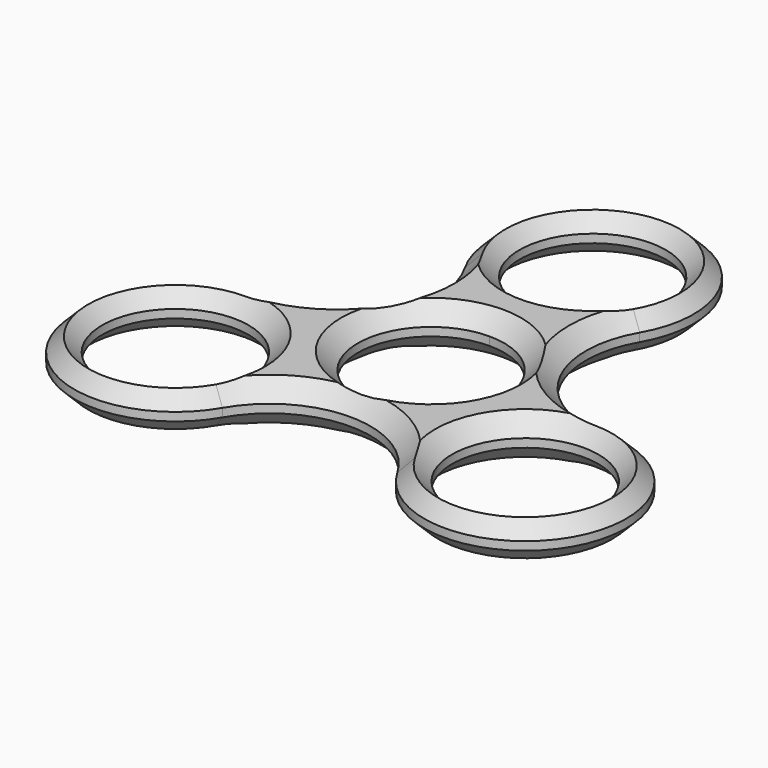
from build123d import *

# Parameters (mm, degrees)
F0_R         = 11.049
F1_DEPTH     = 6.35
F2_T2_ANGLE  = 120
F2_T4_ANGLE  = 240
F2_T6_ANGLE  = 120
F2_T8_ANGLE  = 240
F2_T10_ANGLE = 120
F2_T12_ANGLE = 240
F2_T22_ANGLE = 120
F2_T24_ANGLE = 240
F2_T26_ANGLE = 120
F2_T28_ANGLE = 240
F2_T30_ANGLE = 120
F2_T32_ANGLE = 240


# Not quite as in the source:
# - a fillet or chamfer that OpenCascade refuses, or shapes differently, is made with other operations: its cross-section is extruded or revolved along the edge and cut away or added


with BuildPart() as f1:
    # F0 (on Top) → F1 (new body)
    with BuildSketch(Plane.XY):
        with BuildLine():
            ThreePointArc((26.3964543073, 0), (13.1982271537, 7.62), (13.1982271537, 22.86))
            ThreePointArc((13.1982271537, 22.86), (0, 45.72), (-13.1982271537, 22.86))
            ThreePointArc((-13.1982271537, 22.86), (-13.1982271537, 7.62), (-26.3964543073, 0))
            ThreePointArc((-26.3964543073, 0), (-39.594681461, -22.86), (-13.1982271537, -22.86))
            ThreePointArc((-13.1982271537, -22.86), (0, -15.24), (13.1982271537, -22.86))
            ThreePointArc((13.1982271537, -22.86), (39.594681461, -22.86), (26.3964543073, 0))
        make_face()
        with Locations((-26.3964543073, -15.24)):
            Circle(F0_R, mode=Mode.SUBTRACT)
        with Locations((26.3964543073, -15.24)):
            Circle(F0_R, mode=Mode.SUBTRACT)
        with BuildLine():
            ThreePointArc((0, 11.049), (7.8128228253, 7.8128228253), (11.049, 0))
            ThreePointArc((11.049, 0), (-7.8128228253, -7.8128228253), (0, 11.049))
        make_face(mode=Mode.SUBTRACT)
        with Locations((0, 30.48)):
            Circle(F0_R, mode=Mode.SUBTRACT)
    extrude(amount=F1_DEPTH)

    # F2: chamfer of 2.54 on 20 edges, made by hand

    # F2_s1 → F2_t2 (revolve, cut)
    with BuildSketch(Plane.YZ.offset(26.3964543073)):
        Polygon((0, 3.81), (-2.54, 6.35), (0, 6.35), align=None)
    revolve(axis=Axis((26.3964543073, 15.24, 6.35), (0, 0, -1)), revolution_arc=F2_T2_ANGLE, mode=Mode.SUBTRACT)

    # F2_s3 → F2_t4 (revolve, cut)
    with BuildSketch(Plane(origin=(13.1982271537, 22.86, 0), x_dir=(0, 0, 1), z_dir=(-0.5, -0.8660254038, 0))):
        Polygon((6.35, 2.54), (3.81, 0), (6.35, 0), align=None)
    revolve(axis=Axis((0, 30.48, 6.35), (0, 0, 1)), revolution_arc=F2_T4_ANGLE, mode=Mode.SUBTRACT)

    # F2_s5 → F2_t6 (revolve, cut)
    with BuildSketch(Plane(origin=(-13.1982271537, 22.86, 0), x_dir=(0, 0, 1), z_dir=(-0.5, 0.8660254038, 0))):
        Polygon((6.35, 2.54), (3.81, 0), (6.35, 0), align=None)
    revolve(axis=Axis((-26.3964543073, 15.24, 6.35), (0, 0, -1)), revolution_arc=F2_T6_ANGLE, mode=Mode.SUBTRACT)

    # F2_s7 → F2_t8 (revolve, cut)
    with BuildSketch(Plane.YZ.offset(-26.3964543073)):
        Polygon((-2.54, 6.35), (0, 3.81), (0, 6.35), align=None)
    revolve(axis=Axis((-26.3964543073, -15.24, 6.35), (0, 0, 1)), revolution_arc=F2_T8_ANGLE, mode=Mode.SUBTRACT)

    # F2_s9 → F2_t10 (revolve, cut)
    with BuildSketch(Plane(origin=(-13.1982271537, -22.86, 0), x_dir=(0, 0, 1), z_dir=(-0.5, -0.8660254038, 0))):
        Polygon((6.35, 2.54), (3.81, 0), (6.35, 0), align=None)
    revolve(axis=Axis((0, -30.48, 6.35), (0, 0, -1)), revolution_arc=F2_T10_ANGLE, mode=Mode.SUBTRACT)

    # F2_s11 → F2_t12 (revolve, cut)
    with BuildSketch(Plane(origin=(13.1982271537, -22.86, 0), x_dir=(0, 0, 1), z_dir=(-0.5, 0.8660254038, 0))):
        Polygon((6.35, 2.54), (3.81, 0), (6.35, 0), align=None)
    revolve(axis=Axis((26.3964543073, -15.24, 6.35), (0, 0, 1)), revolution_arc=F2_T12_ANGLE, mode=Mode.SUBTRACT)

    # F2_s13 → F2_t14 (revolve, cut)
    with BuildSketch(Plane.XZ.offset(15.24)):
        Polygon((-12.8074543073, 6.35), (-15.3474543073, 3.81), (-15.3474543073, 6.35), align=None)
    revolve(axis=Axis((-26.3964543073, -15.24, 6.35), (0, 0, 1)), mode=Mode.SUBTRACT)

    # F2_s15 → F2_t16 (revolve, cut)
    with BuildSketch(Plane.XZ.offset(15.24)):
        Polygon((39.9854543073, 6.35), (37.4454543073, 3.81), (37.4454543073, 6.35), align=None)
    revolve(axis=Axis((26.3964543073, -15.24, 6.35), (0, 0, 1)), mode=Mode.SUBTRACT)

    # F2_s17 → F2_t18 (revolve, cut)
    with BuildSketch(Plane.YZ):
        Polygon((13.589, 6.35), (11.049, 3.81), (11.049, 6.35), align=None)
    revolve(axis=Axis((0, 0, 6.35), (0, 0, 1)), mode=Mode.SUBTRACT)

    # F2_s19 → F2_t20 (revolve, cut)
    with BuildSketch(Plane.XZ.offset(-30.48)):
        Polygon((13.589, 6.35), (11.049, 3.81), (11.049, 6.35), align=None)
    revolve(axis=Axis((0, 30.48, 6.35), (0, 0, 1)), mode=Mode.SUBTRACT)

    # F2_s21 → F2_t22 (revolve, cut)
    with BuildSketch(Plane.YZ.offset(26.3964543073)):
        Polygon((0, 2.54), (-2.54, 0), (0, 0), align=None)
    revolve(axis=Axis((26.3964543073, 15.24, 0), (0, 0, -1)), revolution_arc=F2_T22_ANGLE, mode=Mode.SUBTRACT)

    # F2_s23 → F2_t24 (revolve, cut)
    with BuildSketch(Plane(origin=(13.1982271537, 22.86, 0), x_dir=(0, 0, 1), z_dir=(-0.5, -0.8660254038, 0))):
        Polygon((0, 2.54), (2.54, 0), (0, 0), align=None)
    revolve(axis=Axis((0, 30.48, 0), (0, 0, 1)), revolution_arc=F2_T24_ANGLE, mode=Mode.SUBTRACT)

    # F2_s25 → F2_t26 (revolve, cut)
    with BuildSketch(Plane(origin=(-13.1982271537, 22.86, 0), x_dir=(0, 0, 1), z_dir=(-0.5, 0.8660254038, 0))):
        Polygon((2.54, 0), (0, 2.54), (0, 0), align=None)
    revolve(axis=Axis((-26.3964543073, 15.24, 0), (0, 0, -1)), revolution_arc=F2_T26_ANGLE, mode=Mode.SUBTRACT)

    # F2_s27 → F2_t28 (revolve, cut)
    with BuildSketch(Plane.YZ.offset(-26.3964543073)):
        Polygon((0, 2.54), (-2.54, 0), (0, 0), align=None)
    revolve(axis=Axis((-26.3964543073, -15.24, 0), (0, 0, 1)), revolution_arc=F2_T28_ANGLE, mode=Mode.SUBTRACT)

    # F2_s29 → F2_t30 (revolve, cut)
    with BuildSketch(Plane(origin=(-13.1982271537, -22.86, 0), x_dir=(0, 0, 1), z_dir=(-0.5, -0.8660254038, 0))):
        Polygon((2.54, 0), (0, 2.54), (0, 0), align=None)
    revolve(axis=Axis((0, -30.48, 0), (0, 0, -1)), revolution_arc=F2_T30_ANGLE, mode=Mode.SUBTRACT)

    # F2_s31 → F2_t32 (revolve, cut)
    with BuildSketch(Plane(origin=(13.1982271537, -22.86, 0), x_dir=(0, 0, 1), z_dir=(-0.5, 0.8660254038, 0))):
        Polygon((0, 2.54), (2.54, 0), (0, 0), align=None)
    revolve(axis=Axis((26.3964543073, -15.24, 0), (0, 0, 1)), revolution_arc=F2_T32_ANGLE, mode=Mode.SUBTRACT)

    # F2_s33 → F2_t34 (revolve, cut)
    with BuildSketch(Plane.XZ.offset(15.24)):
        Polygon((-15.3474543073, 2.54), (-12.8074543073, 0), (-15.3474543073, 0), align=None)
    revolve(axis=Axis((-26.3964543073, -15.24, 0), (0, 0, 1)), mode=Mode.SUBTRACT)

    # F2_s35 → F2_t36 (revolve, cut)
    with BuildSketch(Plane.XZ.offset(15.24)):
        Polygon((37.4454543073, 2.54), (39.9854543073, 0), (37.4454543073, 0), align=None)
    revolve(axis=Axis((26.3964543073, -15.24, 0), (0, 0, 1)), mode=Mode.SUBTRACT)

    # F2_s37 → F2_t38 (revolve, cut)
    with BuildSketch(Plane.YZ):
        Polygon((11.049, 2.54), (13.589, 0), (11.049, 0), align=None)
    revolve(axis=Axis((0, 0, 0), (0, 0, -1)), mode=Mode.SUBTRACT)

    # F2_s39 → F2_t40 (revolve, cut)
    with BuildSketch(Plane.XZ.offset(-30.48)):
        Polygon((11.049, 2.54), (13.589, 0), (11.049, 0), align=None)
    revolve(axis=Axis((0, 30.48, 0), (0, 0, 1)), mode=Mode.SUBTRACT)


solid = f1.part
